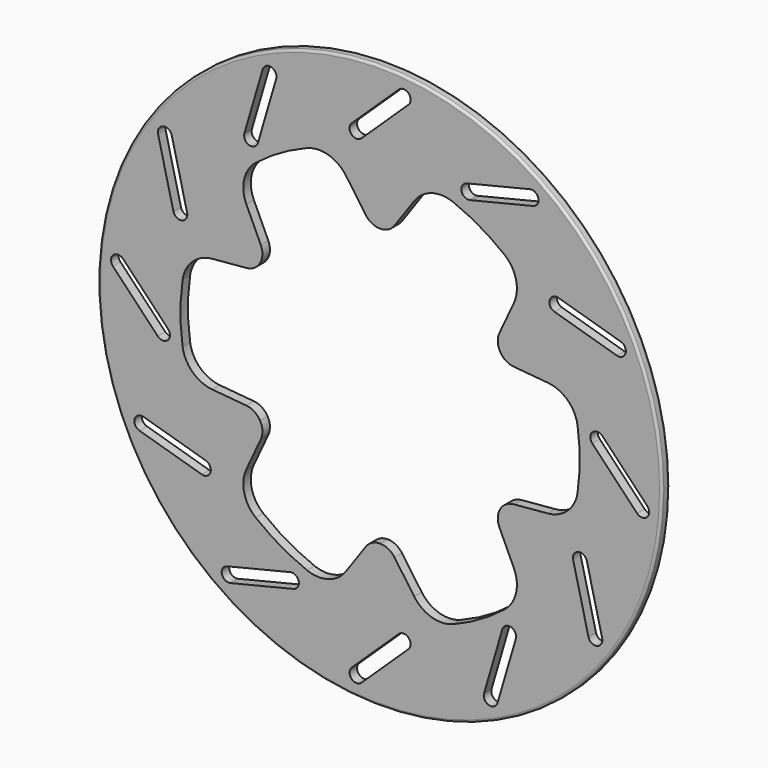
from build123d import *

# Parameters (mm, degrees)
F0_R     = 120
F1_DEPTH = 4
F2_R     = 1
F3_R     = 1


# Not quite as in the source:
# - ends of sketch curves that miss each other by under 0.0002 mm in the source are joined


with BuildPart() as f1:
    # F0 (on Front) → F1 (new body)
    with BuildSketch(Plane.XZ):
        with Locations((0.769432, 5.271099)):
            Circle(F0_R)
        with BuildLine():
            ThreePointArc((-62.9582121085, -89.2513825538), (-66.5821895538, -87.0453028915), (-64.3761098915, -83.4213254462))
            Line((-64.3761098915, -83.4213254462), (-37.509664, -76.887277))
            ThreePointArc((-37.509664, -76.887277), (-33.8856864462, -79.0933561085), (-36.0917661085, -82.7173335538))
            Line((-36.0917661085, -82.7173335538), (-62.9582121085, -89.2513825538))
        make_face(mode=Mode.SUBTRACT)
        with BuildLine():
            ThreePointArc((-101.6815671027, -44.7239493504), (-103.7169843504, -41.0014398973), (-99.9944748973, -38.9660226496))
            Line((-99.9944748973, -38.9660226496), (-73.460425, -46.740593))
            ThreePointArc((-73.460425, -46.740593), (-71.4250076496, -50.4631031027), (-75.1475171027, -52.4985203504))
            Line((-75.1475171027, -52.4985203504), (-101.6815671027, -44.7239493504))
        make_face(mode=Mode.SUBTRACT)
        with BuildLine():
            ThreePointArc((-112.9532601885, 13.1996168201), (-112.8547281799, 17.4411131885), (-108.6132318115, 17.3425811799))
            Line((-108.6132318115, 17.3425811799), (-89.521356, -2.657419))
            ThreePointArc((-89.521356, -2.657419), (-89.6198878201, -6.8989151885), (-93.8613841885, -6.8003831799))
            Line((-93.8613841885, -6.8003831799), (-112.9532601885, 13.1996168201))
        make_face(mode=Mode.SUBTRACT)
        with BuildLine():
            ThreePointArc((-7.1590858201, -108.4515931885), (-11.4005821885, -108.3530611799), (-11.3020501799, -104.1115648115))
            Line((-11.3020501799, -104.1115648115), (8.69795, -85.019689))
            ThreePointArc((8.69795, -85.019689), (12.9394461885, -85.1182218201), (12.8409141799, -89.3597181885))
            Line((12.8409141799, -89.3597181885), (-7.1590858201, -108.4515931885))
        make_face(mode=Mode.SUBTRACT)
        with BuildLine():
            ThreePointArc((50.7644803504, -97.1799001027), (47.0419708973, -99.2153173504), (45.0065536496, -95.4928078973))
            Line((45.0065536496, -95.4928078973), (52.781124, -68.958759))
            ThreePointArc((52.781124, -68.958759), (56.5036341027, -66.9233416496), (58.5390513504, -70.6458511027))
            Line((58.5390513504, -70.6458511027), (50.7644803504, -97.1799001027))
        make_face(mode=Mode.SUBTRACT)
        with BuildLine():
            ThreePointArc((95.2919145538, -58.4565451085), (93.0858348915, -62.0805225538), (89.4618574462, -59.8744428915))
            Line((89.4618574462, -59.8744428915), (82.927808, -33.007997))
            ThreePointArc((82.927808, -33.007997), (85.1338871085, -29.3840194462), (88.7578645538, -31.5900991085))
            Line((88.7578645538, -31.5900991085), (95.2919145538, -58.4565451085))
        make_face(mode=Mode.SUBTRACT)
        with BuildLine():
            ThreePointArc((114.4921251885, -2.6574188201), (114.3935931799, -6.8989151885), (110.1520968115, -6.8003831799))
            Line((110.1520968115, -6.8003831799), (91.060221, 13.199617))
            ThreePointArc((91.060221, 13.199617), (91.1587528201, 17.4411131885), (95.4002491885, 17.3425811799))
            Line((95.4002491885, 17.3425811799), (114.4921251885, -2.6574188201))
        make_face(mode=Mode.SUBTRACT)
        with BuildLine():
            ThreePointArc((-93.7530495538, 68.9987431085), (-91.5469698915, 72.6227205538), (-87.9229924462, 70.4166408915))
            Line((-87.9229924462, 70.4166408915), (-81.388943, 43.550195))
            ThreePointArc((-81.388943, 43.550195), (-83.5950221085, 39.9262174462), (-87.2189995538, 42.1322971085))
            Line((-87.2189995538, 42.1322971085), (-93.7530495538, 68.9987431085))
        make_face(mode=Mode.SUBTRACT)
        with BuildLine():
            ThreePointArc((-49.2256163504, 107.7220981027), (-45.5031068973, 109.7575153504), (-43.4676896496, 106.0350058973))
            Line((-43.4676896496, 106.0350058973), (-51.24226, 79.500956))
            ThreePointArc((-51.24226, 79.500956), (-54.9647691027, 77.4655396496), (-57.0001863504, 81.1880491027))
            Line((-57.0001863504, 81.1880491027), (-49.2256163504, 107.7220981027))
        make_face(mode=Mode.SUBTRACT)
        with BuildLine():
            ThreePointArc((15.296097835, 79.396963116), (22.7229925826, 84.7551105395), (31.8731110928, 84.3758472359))
            ThreePointArc((31.8731110928, 84.3758472359), (43.2694321028, 78.8832582623), (53.724314001, 71.7600490012))
            ThreePointArc((53.724314001, 71.7600490012), (58.6278254217, 64.0254452963), (57.7009806311, 54.9144921712))
            Line((57.7009806311, 54.9144921712), (51.557275, 41.678832))
            ThreePointArc((51.557275, 41.678832), (50.8675495212, 38.1873960638), (51.8649313537, 34.7710992042))
            ThreePointArc((51.8649313537, 34.7710992042), (54.3248400002, 32.1991927067), (57.6933760416, 31.0507944662))
            Line((57.6933760416, 31.0507944662), (72.227646, 29.753569))
            ThreePointArc((72.227646, 29.753569), (80.5813855597, 26.0007639127), (84.8279934344, 17.8868970652))
            ThreePointArc((84.8279934344, 17.8868970652), (85.769432, 5.271099), (84.8279927873, -7.3446989681))
            ThreePointArc((84.8279927873, -7.3446989681), (80.5813855597, -15.4585659127), (72.2276460446, -19.2113714997))
            Line((72.2276460446, -19.2113714997), (57.693376, -20.508597))
            ThreePointArc((57.693376, -20.508597), (54.3248400002, -21.6569947067), (51.8649313537, -24.2289012042))
            ThreePointArc((51.8649313537, -24.2289012042), (50.8675495212, -27.6451980638), (51.5572758618, -31.1366350642))
            Line((51.5572758618, -31.1366350642), (57.700981, -44.372294))
            ThreePointArc((57.700981, -44.372294), (58.6278254217, -53.4832472963), (53.7243149172, -61.217850896))
            ThreePointArc((53.7243149172, -61.217850896), (43.2694321028, -68.3410602623), (31.8731109925, -73.833648981))
            ThreePointArc((31.8731109925, -73.833648981), (22.7229925826, -74.2129125395), (15.296097835, -68.854765116))
            Line((15.296097835, -68.854765116), (6.905533, -56.91633))
            ThreePointArc((6.905533, -56.91633), (4.2267227516, -54.5732912865), (0.769432, -53.728901))
            ThreePointArc((0.769432, -53.728901), (-2.6878587516, -54.5732912865), (-5.3666687757, -56.9163301576))
            Line((-5.3666687757, -56.9163301576), (-13.757233, -68.854765))
            ThreePointArc((-13.757233, -68.854765), (-21.1841275826, -74.2129125395), (-30.3342460928, -73.8336492359))
            ThreePointArc((-30.3342460928, -73.8336492359), (-41.7305681028, -68.3410602623), (-52.185450001, -61.2178510012))
            ThreePointArc((-52.185450001, -61.2178510012), (-57.0889604217, -53.4832472963), (-56.1621156311, -44.3722941712))
            Line((-56.1621156311, -44.3722941712), (-50.018411, -31.136635))
            ThreePointArc((-50.018411, -31.136635), (-49.3286845212, -27.6451980638), (-50.3260663537, -24.2289012042))
            ThreePointArc((-50.3260663537, -24.2289012042), (-52.7859750002, -21.6569947067), (-56.1545110416, -20.5085964662))
            Line((-56.1545110416, -20.5085964662), (-70.688781, -19.211372))
            ThreePointArc((-70.688781, -19.211372), (-79.0425205597, -15.4585659127), (-83.2891284344, -7.3446990652))
            ThreePointArc((-83.2891284344, -7.3446990652), (-84.230568, 5.271099), (-83.2891287873, 17.8868969681))
            ThreePointArc((-83.2891287873, 17.8868969681), (-79.0425205597, 26.0007639127), (-70.6887810446, 29.7535694997))
            Line((-70.6887810446, 29.7535694997), (-56.154511, 31.050794))
            ThreePointArc((-56.154511, 31.050794), (-52.7859750002, 32.1991927067), (-50.3260663537, 34.7710992042))
            ThreePointArc((-50.3260663537, 34.7710992042), (-49.3286845212, 38.1873960638), (-50.0184108618, 41.6788330642))
            Line((-50.0184108618, 41.6788330642), (-56.162116, 54.914492))
            ThreePointArc((-56.162116, 54.914492), (-57.0889604217, 64.0254452963), (-52.1854499172, 71.760048896))
            ThreePointArc((-52.1854499172, 71.760048896), (-41.7305681028, 78.8832582623), (-30.3342469925, 84.375846981))
            ThreePointArc((-30.3342469925, 84.375846981), (-21.1841275826, 84.7551105395), (-13.757232835, 79.396963116))
            Line((-13.757232835, 79.396963116), (-5.366668, 67.458528))
            ThreePointArc((-5.366668, 67.458528), (-2.6878587516, 65.1154892865), (0.769432, 64.271099))
            ThreePointArc((0.769432, 64.271099), (4.2267227516, 65.1154892865), (6.9055327757, 67.4585281576))
            Line((6.9055327757, 67.4585281576), (15.296097835, 79.396963116))
        make_face(mode=Mode.SUBTRACT)
        with BuildLine():
            ThreePointArc((103.2204321027, 55.2661473504), (105.2558493504, 51.5436378973), (101.5333398973, 49.5082206496))
            Line((101.5333398973, 49.5082206496), (74.99929, 57.282791))
            ThreePointArc((74.99929, 57.282791), (72.9638726496, 61.0053001027), (76.6863821027, 63.0407173504))
            Line((76.6863821027, 63.0407173504), (103.2204321027, 55.2661473504))
        make_face(mode=Mode.SUBTRACT)
        with BuildLine():
            ThreePointArc((64.4970771085, 99.7935805538), (68.1210545538, 97.5875008915), (65.9149748915, 93.9635234462))
            Line((65.9149748915, 93.9635234462), (39.048529, 87.429474))
            ThreePointArc((39.048529, 87.429474), (35.4245514462, 89.6355541085), (37.6306311085, 93.2595315538))
            Line((37.6306311085, 93.2595315538), (64.4970771085, 99.7935805538))
        make_face(mode=Mode.SUBTRACT)
        with BuildLine():
            ThreePointArc((8.6979498201, 118.9937911885), (12.9394461885, 118.8952591799), (12.8409141799, 114.6537628115))
            Line((12.8409141799, 114.6537628115), (-7.159085, 95.561887))
            ThreePointArc((-7.159085, 95.561887), (-11.4005821885, 95.6604188201), (-11.3020501799, 99.9019151885))
            Line((-11.3020501799, 99.9019151885), (8.6979498201, 118.9937911885))
        make_face(mode=Mode.SUBTRACT)
    extrude(amount=F1_DEPTH)

    # F2
    f2_edges = [f1.edges().sort_by_distance(p)[0] for p in [
        (-119.230568, -4, 5.271099),
    ]]
    fillet(f2_edges, radius=F2_R)

    # F3
    f3_edges = [f1.edges().sort_by_distance(p)[0] for p in [
        (-119.230568, 0, 5.271099),
    ]]
    fillet(f3_edges, radius=F3_R)


solid = f1.part
